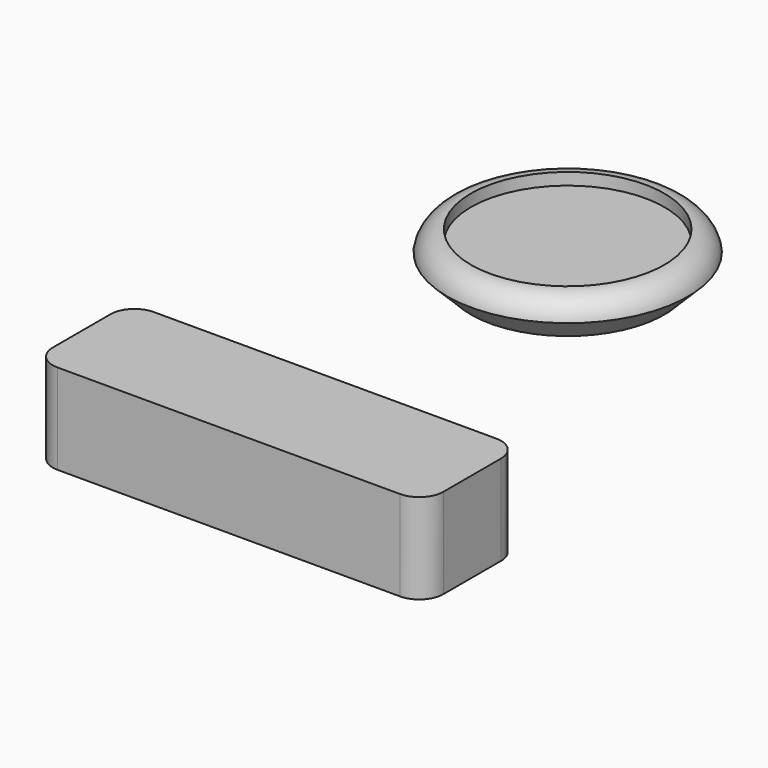
from build123d import *

# Parameters (mm, degrees)
F0_W     = 82.55
F0_H     = 19.05
F1_DEPTH = 12.7
F3_R     = 5.08
F4_R     = 5.08
F6_DEPTH = 2.54


# Not quite as in the source:
# - a fillet or chamfer that OpenCascade refuses, or shapes differently, is made with other operations: its cross-section is extruded or revolved along the edge and cut away or added


with BuildPart() as f1:
    # F0 (on Front) → F1 (new body, symmetric)
    with BuildSketch(Plane.XZ):
        Rectangle(F0_W, F0_H)
    extrude(amount=F1_DEPTH, both=True)

    # F3
    f3_edges = [f1.edges().sort_by_distance(p)[0] for p in [
        (-41.275, -12.7, 0),
        (41.275, -12.7, 0),
        (41.275, 12.7, 0),
        (-41.275, 12.7, 0),
    ]]
    fillet(f3_edges, radius=F3_R)


with BuildPart() as f2:
    # F0 (on Front) → F2 (revolve)
    with BuildSketch(Plane.XZ):
        Polygon((35.9360538423, 61.8671737611), (35.9360538423, 52.5995560322), (50.8114657512, 52.5995560322), (61.4588148892, 52.5995560322), (61.4588148892, 61.8671737611), align=None)
    revolve(axis=Axis((61.4588148892, 0, 54.2103461921), (0, 0, -1)))

    # F4
    f4_edges = [f2.edges().sort_by_distance(p)[0] for p in [
        (86.981576, 0, 61.867174),
    ]]
    fillet(f4_edges, radius=F4_R)

    # F5: chamfer of 5.08 on 1 edges, made by hand

    # F5_s1 → F5_t2 (revolve, cut)
    with BuildSketch(Plane.XZ):
        Polygon((35.9360538423, 57.6795560322), (41.0160538423, 52.5995560322), (35.9360538423, 52.5995560322), align=None)
    revolve(axis=Axis((61.4588148892, 0, 52.5995560322), (0, 0, -1)), mode=Mode.SUBTRACT)

    # F6 (cut): a face of the model
    f6_faces = [f2.faces().sort_by_distance(p)[0] for p in [
        (61.4588148892, 0, 61.8671737611),
    ]]
    extrude(f6_faces, amount=-F6_DEPTH, mode=Mode.SUBTRACT)


solid = Compound([f1.part, f2.part])
